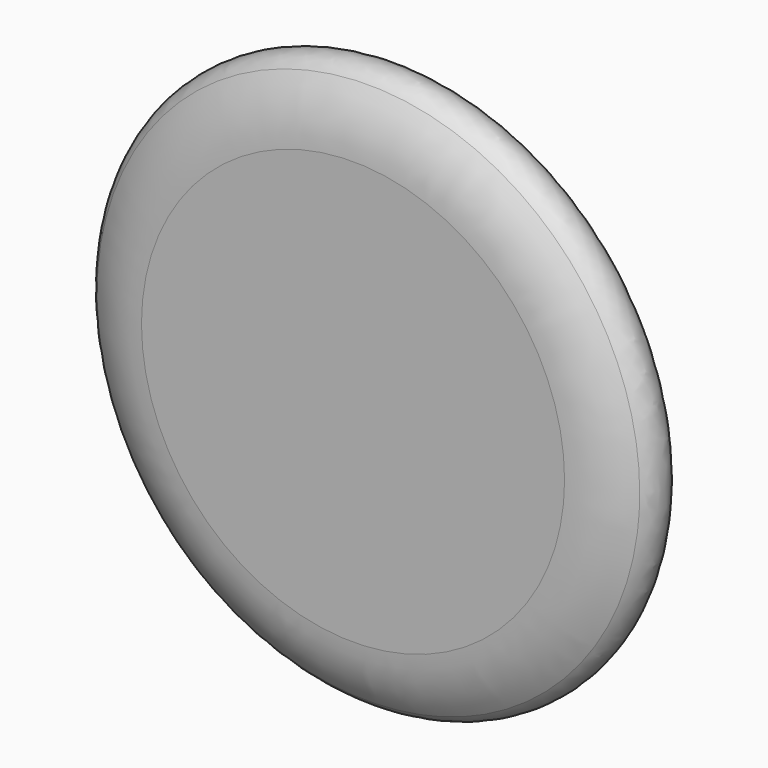
from build123d import *

# Parameters (mm, degrees)
F2_R     = 124.464334162
F3_DEPTH = 25.4
F5_R     = 9.6970890036
F6_T     = 2.54


# Not quite as in the source:
# - a fillet or chamfer that OpenCascade refuses, or shapes differently, is made with other operations: its cross-section is extruded or revolved along the edge and cut away or added
# - a shell that OpenCascade refuses in one call is made with other operations: the cavity is built on its own and cut out


with BuildPart() as f3:
    # F2 (on Front) → F3 (new body)
    with BuildSketch(Plane.XZ):
        Circle(F2_R)
    extrude(amount=F3_DEPTH)

    # F4: fillet of radius 41.6982966493 on 1 edges, made by hand

    # F4_s1 → F4_t2 (revolve, cut)
    with BuildSketch(Plane.XY):
        with BuildLine():
            ThreePointArc((124.464334162, 0), (109.0955263093, -18.4749628471), (86.0831738123, -25.4))
            Line((86.0831738123, -25.4), (124.464334162, -25.4))
            Line((124.464334162, -25.4), (124.464334162, 0))
        make_face()
    revolve(axis=Axis((0, -25.4, 0), (0, -1, 0)), mode=Mode.SUBTRACT)

    # F5
    f5_edges = [f3.edges().sort_by_distance(p)[0] for p in [
        (-124.464334, 0, 0),
    ]]
    fillet(f5_edges, radius=F5_R)

    # F6: shell of thickness 2.54, made by hand


with BuildPart() as f6_core1:
    # F6_t2: copy of F3
    add(f3.part)

    # the walls: a layer under each face that stays
    f6_faces = [f6_core1.faces().sort_by_distance(p)[0] for p in [
        (-113.9773406634, -6.7265898841, 0),
        (-98.8565693577, -23.3953843301, 0),
        (0, -25.4, 0),
    ]]
    thicken(f6_faces, amount=-F6_T, mode=Mode.SUBTRACT)


with BuildPart() as f3_1:
    add(f3.part)

    # what is left inside the walls is the cavity
    f6_cavity = [f6_core1.part.solids().sort_by_distance(p)[0] for p in [
        (0, -0.0254, -39.133226),
    ]]
    add(f6_cavity, mode=Mode.SUBTRACT)


solid = f3_1.part
